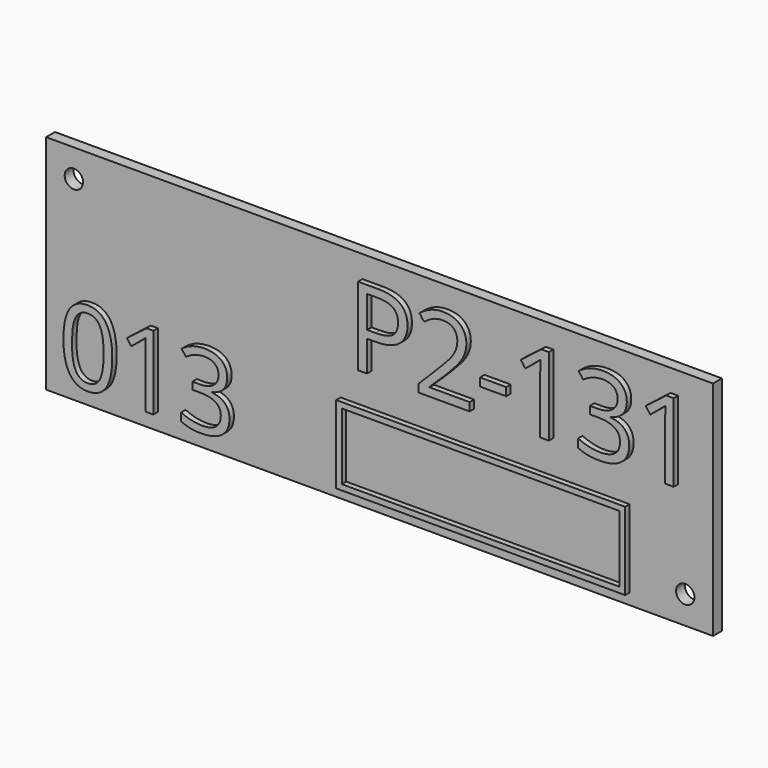
from build123d import *

# Parameters (mm, degrees)
F0_W         = 120
F0_H         = 40
F1_DEPTH     = 2
F3_D         = 3.3
F4_TEXT_SIZE = 19.654007575
F5_DEPTH     = 1
F6_TEXT_SIZE = 18.5894526641
F7_DEPTH     = 1
F8_W         = 52
F8_H         = 14
F8_W_2       = 49.99999962
F8_H_2       = 11.99999962
F9_DEPTH     = 1


# Not quite as in the source:
# - Text() gives the source's letters only with a copy of the font that has no kerning and outlines rounded to 1/6400 em; it was checked with that copy


with BuildPart() as f1:
    # F0 (on Front) → F1 (new body)
    with BuildSketch(Plane.XZ):
        Rectangle(F0_W, F0_H)
    extrude(amount=F1_DEPTH)

    # F3 (through all)
    with Locations(Plane.XZ.offset(2)):
        with Locations((-55, 15), (55, -15)):
            Hole(F3_D / 2)

    # F4 (on face) → F5 (join)
    with BuildSketch(Plane.XZ.offset(2)):
        with Locations((-5, 2)):
            Text('P2-131', F4_TEXT_SIZE, font='Open Sans', text_align=(TextAlign.LEFT, TextAlign.BOTTOM))
    extrude(amount=F5_DEPTH)

    # F6 (on face) → F7 (join)
    with BuildSketch(Plane.XZ.offset(2)):
        with Locations((-57, -17)):
            Text('013', F6_TEXT_SIZE, font='Open Sans', text_align=(TextAlign.LEFT, TextAlign.BOTTOM))
    extrude(amount=F7_DEPTH)

    # F8 (on face) → F9 (join)
    with BuildSketch(Plane.XZ.offset(2)):
        with Locations((19, -11)):
            Rectangle(F8_W, F8_H)
        with Locations((19, -11)):
            Rectangle(F8_W_2, F8_H_2, mode=Mode.SUBTRACT)
    extrude(amount=F9_DEPTH)


solid = f1.part
